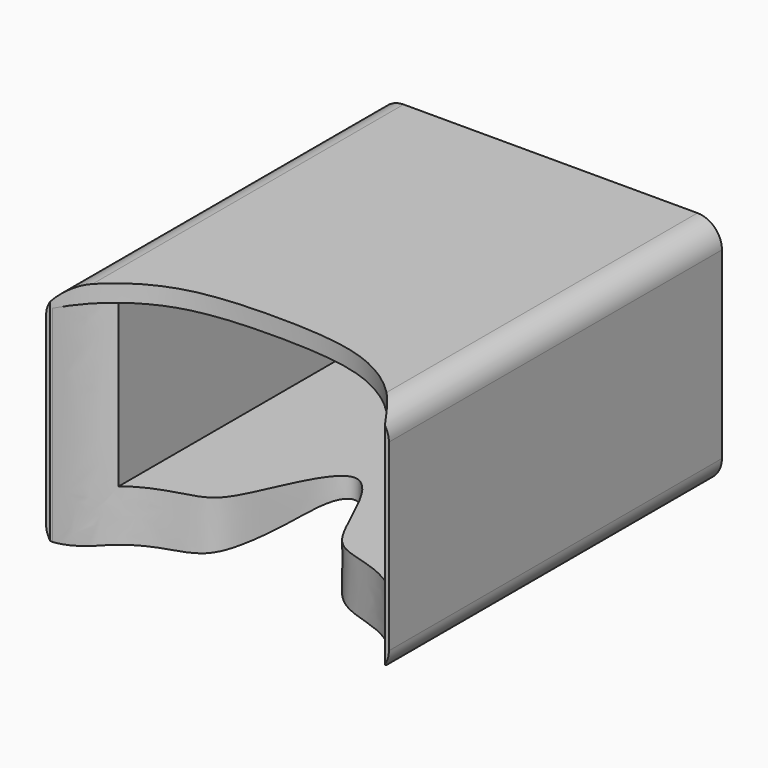
from build123d import *

# Parameters (mm, degrees)
F0_W      = 140
F0_H      = 170
F1_DEPTH  = 95
F2_W      = 110
F2_H      = 67
F3_DEPTH  = 170.001
F5_DEPTH  = 88
F7_DEPTH  = 95.001
F8_R      = 10
F10_DEPTH = 170.001


with BuildPart() as f1:
    # F0 (on Top) → F1 (new body)
    with BuildSketch(Plane.XY):
        Rectangle(F0_W, F0_H)
    extrude(amount=F1_DEPTH)

    # F2 (on face) → F3 (cut, through all)
    with BuildSketch(Plane.XZ.offset(85)):
        with Locations((0, 54.5)):
            Rectangle(F2_W, F2_H)
    extrude(amount=-F3_DEPTH, mode=Mode.SUBTRACT)

    # F4 (on face) → F5 (cut)
    with BuildSketch(Plane(origin=(0, 0, 0), x_dir=(1, 0, 0), z_dir=(0, 0, -1))):
        with BuildLine():
            add(Edge.make_bspline(
                [(0, 15), (-7.79441, 15), (-19.466411, 48.056936), (-30.975012, 59.107625), (-57.856268, 61.12551), (-68.258241, 85)],
                knots=[0, 0, 0, 0, 0.355883, 0.597297, 1, 1, 1, 1], degree=3))
            add(Edge.make_bspline(
                [(0, 15), (7.79441, 15), (19.466411, 48.056936), (30.975012, 59.107625), (57.856268, 61.12551), (68.258241, 85)],
                knots=[0, 0, 0, 0, 0.355883, 0.597297, 1, 1, 1, 1], degree=3))
            Line((68.258241, 85), (-68.258241, 85))
        make_face()
    extrude(amount=-F5_DEPTH, mode=Mode.SUBTRACT)

    # F6 (on face) → F7 (cut, through all)
    with BuildSketch(Plane.XY.offset(95)):
        with BuildLine():
            add(Edge.make_bspline(
                [(0, -55), (25.389496, -55), (47.041007, -60.614282), (62.843867, -75.413413), (68.355819, -85)],
                knots=[0, 0, 0, 0, 0.564508, 1, 1, 1, 1], degree=3))
            add(Edge.make_bspline(
                [(0, -55), (-25.389496, -55), (-47.041007, -60.614282), (-62.843867, -75.413413), (-68.355819, -85)],
                knots=[0, 0, 0, 0, 0.564508, 1, 1, 1, 1], degree=3))
            Line((-68.355819, -85), (68.355819, -85))
        make_face()
    extrude(amount=-F7_DEPTH, mode=Mode.SUBTRACT)

    # F8
    f8_edges = [f1.edges().sort_by_distance(p)[0] for p in [
        (70, 0, 95),
        (70, 0, 0),
        (-70, 0, 0),
        (-70, 0, 95),
    ]]
    fillet(f8_edges, radius=F8_R)

    # F9 (on face) → F10 (cut, through all)
    with BuildSketch(Plane(origin=(0, 85, 0), x_dir=(-1, 0, 0), z_dir=(0, 1, 0))):
        with BuildLine():
            add(Edge.make_bspline(
                [(0, 13), (14.179069, 13), (11.016984, 0), (40, 0)],
                knots=[0, 0, 0, 0, 42.059482, 42.059482, 42.059482, 42.059482], degree=3))
            add(Edge.make_bspline(
                [(0, 13), (-14.179069, 13), (-11.016984, 0), (-40, 0)],
                knots=[0, 0, 0, 0, 42.059482, 42.059482, 42.059482, 42.059482], degree=3))
            Line((-40, 0), (40, 0))
        make_face()
    extrude(amount=-F10_DEPTH, mode=Mode.SUBTRACT)


solid = f1.part
